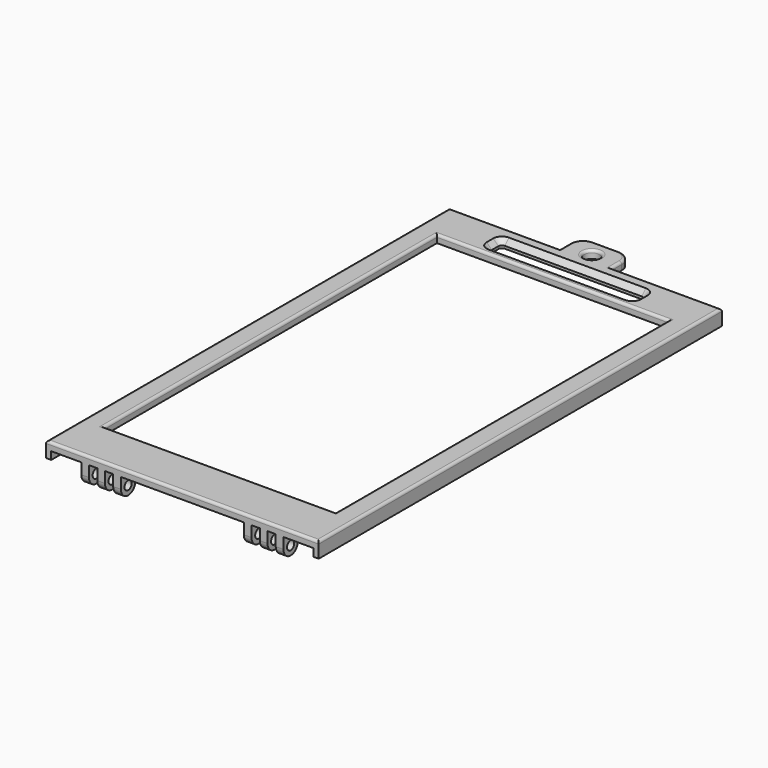
from build123d import *

# Parameters (mm, degrees)
F0_W         = 106
F0_H         = 188.5
F0_W_2       = 90
F0_H_2       = 161.75
F0_H_3       = 7.5
F1_DEPTH     = 3
F2_W         = 3
F2_H         = 7
F3_DEPTH     = 7.75
F4_R         = 3.49999
F5_R         = 1.75
F6_DEPTH     = 86.101
F7_W         = 20
F7_H         = 3
F8_DEPTH     = 10
F9_R         = 3
F10_DEPTH    = 3.001
F11_W        = 2
F11_H        = 196
F12_DEPTH    = 3
F13_R        = 1
F14_R        = 1.75
F15_DEPTH    = 25
F16_T1_DEPTH = 15.5
F16_T4_ANGLE = 90
F16_T6_ANGLE = 90
F18_DEPTH    = 3.0010001
F19_SIZE     = 2


# Not quite as in the source:
# - a fillet or chamfer that OpenCascade refuses, or shapes differently, is made with other operations: its cross-section is extruded or revolved along the edge and cut away or added
# - a fillet or chamfer is up to 0.001 mm smaller than in the source, because OpenCascade refuses the exact size


with BuildPart() as f1:
    # F0 (on Top) → F1 (new body)
    with BuildSketch(Plane.XY):
        with Locations((-16.7186730212, -81.4374315739)):
            Rectangle(F0_W, F0_H)
        with Locations((-16.7186730212, -84.0624315739)):
            Rectangle(F0_W_2, F0_H_2, mode=Mode.SUBTRACT)
        with Locations((-16.7186730212, -179.4374315739)):
            Rectangle(F0_W, F0_H_3)
    extrude(amount=F1_DEPTH)

    # F2 (on face) → F3 (join)
    with BuildSketch(Plane(origin=(0, 0, 0), x_dir=(1, 0, 0), z_dir=(0, 0, -1))):
        with Locations((-48.3186730212, 179.6874315739)):
            Rectangle(F2_W, F2_H)
        with Locations((14.8813269788, 179.6874315739)):
            Rectangle(F2_W, F2_H)
        with Locations((-54.5186730212, 179.6874315739)):
            Rectangle(F2_W, F2_H)
        with Locations((21.0813269788, 179.6874315739)):
            Rectangle(F2_W, F2_H)
        with Locations((-42.1186730212, 179.6874315739)):
            Rectangle(F2_W, F2_H)
        with Locations((8.6813269788, 179.6874315739)):
            Rectangle(F2_W, F2_H)
    extrude(amount=F3_DEPTH)

    # F4 (radius 3.5 in the source; OpenCascade refuses exactly that, so slightly less here)
    f4_edges = [f1.edges().sort_by_distance(p)[0] for p in [
        (-48.318673, -183.187432, -7.75),
        (-48.318673, -176.187432, -7.75),
        (14.881327, -183.187432, -7.75),
        (14.881327, -176.187432, -7.75),
        (-54.518673, -176.187432, -7.75),
        (-54.518673, -183.187432, -7.75),
        (-42.118673, -183.187432, -7.75),
        (-42.118673, -176.187432, -7.75),
        (21.081327, -176.187432, -7.75),
        (8.681327, -176.187432, -7.75),
        (8.681327, -183.187432, -7.75),
        (21.081327, -183.187432, -7.75),
    ]]
    fillet(f4_edges, radius=F4_R)

    # F5 (on face) → F6 (cut, through all)
    with BuildSketch(Plane.YZ.offset(16.3813269788)):
        with Locations((-179.6874315739, -4.25)):
            Circle(F5_R)
    extrude(amount=-F6_DEPTH, mode=Mode.SUBTRACT)

    # F7 (on face) → F8 (join)
    with BuildSketch(Plane(origin=(0, 12.8125684261, 0), x_dir=(-1, 0, 0), z_dir=(0, 1, 0))):
        with Locations((16.7186730212, 1.5)):
            Rectangle(F7_W, F7_H)
    extrude(amount=F8_DEPTH)

    # F9 (on face) → F10 (cut, through all)
    with BuildSketch(Plane(origin=(0, 0, 0), x_dir=(1, 0, 0), z_dir=(0, 0, -1))):
        with Locations((-16.7186730212, -15.8125684261)):
            Circle(F9_R)
    extrude(amount=-F10_DEPTH, mode=Mode.SUBTRACT)

    # F11 (on face) → F12 (join)
    with BuildSketch(Plane(origin=(0, 0, 0), x_dir=(1, 0, 0), z_dir=(0, 0, -1))):
        with Locations((35.2813269788, 85.1874315739)):
            Rectangle(F11_W, F11_H)
        with Locations((-68.7186730212, 85.1874315739)):
            Rectangle(F11_W, F11_H)
    extrude(amount=F12_DEPTH)

    # F13
    f13_edges = [f1.edges().sort_by_distance(p)[0] for p in [
        (14.781327, 12.812568, 3),
        (36.281327, -85.187432, 3),
        (-6.718673, 17.812568, 3),
        (-16.718673, -183.187432, 3),
        (-16.718673, 22.812568, 3),
        (-69.718673, -85.187432, 3),
        (-26.718673, 17.812568, 3),
        (-48.218673, 12.812568, 3),
        (-16.718673, -3.187432, 3),
        (-61.718673, -84.062432, 3),
        (28.281327, -84.062432, 3),
        (-16.718673, -164.937432, 3),
        (-19.718673, 15.812568, 3),
    ]]
    fillet(f13_edges, radius=F13_R)

    # F14 (on face) → F15 (cut)
    with BuildSketch(Plane.YZ.offset(22.5813269788)):
        with Locations((-179.6874315739, -4.25)):
            Circle(F14_R)
    extrude(amount=-F15_DEPTH, mode=Mode.SUBTRACT)

    # F16: fillet of radius 5 on 2 edges, made by hand

    # F16_s2 → F16_t1 (cut)
    with BuildSketch(Plane.XY.offset(-12.5)):
        with BuildLine():
            ThreePointArc((-11.7186730212, 22.8125684261), (-8.1831391152, 21.3481023321), (-6.7186730212, 17.8125684261))
            Line((-6.7186730212, 17.8125684261), (-6.7186730212, 22.8125684261))
            Line((-6.7186730212, 22.8125684261), (-11.7186730212, 22.8125684261))
        make_face()
        with BuildLine():
            ThreePointArc((-26.7186730212, 17.8125684261), (-25.2542069271, 21.3481023321), (-21.7186730212, 22.8125684261))
            Line((-21.7186730212, 22.8125684261), (-26.7186730212, 22.8125684261))
            Line((-26.7186730212, 22.8125684261), (-26.7186730212, 17.8125684261))
        make_face()
    extrude(amount=F16_T1_DEPTH, mode=Mode.SUBTRACT)

    # F16_s3 → F16_t4 (revolve, cut)
    with BuildSketch(Plane.YZ.offset(-21.7186730212)):
        with BuildLine():
            ThreePointArc((21.8125684261, 3), (22.5196752073, 2.7071067812), (22.8125684261, 2))
            Line((22.8125684261, 2), (22.8125684261, 3))
            Line((22.8125684261, 3), (21.8125684261, 3))
        make_face()
    revolve(axis=Axis((-21.7186730212, 17.8125684261, 3), (0, 0, 1)), revolution_arc=F16_T4_ANGLE, mode=Mode.SUBTRACT)

    # F16_s5 → F16_t6 (revolve, cut)
    with BuildSketch(Plane.XZ.offset(-17.8125684261)):
        with BuildLine():
            ThreePointArc((-7.7186730212, 3), (-7.01156624, 2.7071067812), (-6.7186730212, 2))
            Line((-6.7186730212, 2), (-6.7186730212, 3))
            Line((-6.7186730212, 3), (-7.7186730212, 3))
        make_face()
    revolve(axis=Axis((-11.7186730212, 17.8125684261, 3), (0, 0, 1)), revolution_arc=F16_T6_ANGLE, mode=Mode.SUBTRACT)

    # F17 (on face) → F18 (cut, through all)
    with BuildSketch(Plane(origin=(0, 0, 0), x_dir=(1, 0, 0), z_dir=(0, 0, -1))):
        with BuildLine():
            Line((9.8913780288, -0.8125684261), (-43.3287240711, -0.8125684261))
            ThreePointArc((-43.3287240711, -0.8125684261), (-44.3115663992, -1.2196750481), (-44.7186730212, -2.2025173761))
            Line((-44.7186730212, -2.2025173761), (-44.7186730212, -5.4226194761))
            ThreePointArc((-44.7186730212, -5.4226194761), (-44.3115663992, -6.4054618042), (-43.3287240711, -6.8125684261))
            Line((-43.3287240711, -6.8125684261), (9.8913780288, -6.8125684261))
            ThreePointArc((9.8913780288, -6.8125684261), (10.8742203569, -6.4054618042), (11.2813269788, -5.4226194761))
            Line((11.2813269788, -5.4226194761), (11.2813269788, -2.2025173761))
            ThreePointArc((11.2813269788, -2.2025173761), (10.8742203569, -1.2196750481), (9.8913780288, -0.8125684261))
        make_face()
    extrude(amount=-F18_DEPTH, mode=Mode.SUBTRACT)

    # F19
    f19_edges = [f1.edges().sort_by_distance(p)[0] for p in [
        (-16.718673, 6.812568, 3),
    ]]
    chamfer(f19_edges, length=F19_SIZE)


solid = f1.part
